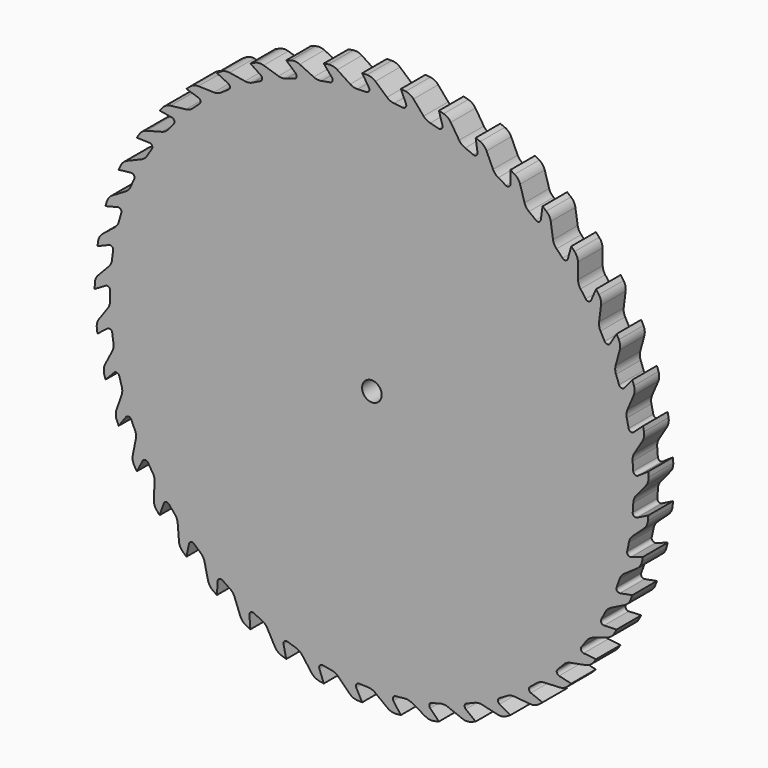
from build123d import *

# Parameters (mm, degrees)
F0_R            = 45
F1_DEPTH        = 5
F4_DEPTH        = 25
F4_COPIES_COUNT = 45
F5_R            = 2
F6_R            = 0.5
F7_R            = 1.5875
F8_DEPTH        = 25


# Not quite as in the source:
# - a pattern or mirror of a feature is missing from the dataset's text; its kind, count and spacing are read off the source's solid


with BuildPart() as f1:
    # F0 (on Front) → F1 (new body)
    with BuildSketch(Plane.XZ):
        Circle(F0_R)
    extrude(amount=F1_DEPTH)

    # F2 (on face) → F4 (cut)
    with BuildSketch(Plane.XZ.offset(5)):
        with BuildLine():
            Line((-6.2627895432, 44.5620630934), (-2.9646501341, 42.396472136))
            ThreePointArc((-2.9646501341, 42.396472136), (-1.4832286099, 42.4741101483), (0, 42.5))
            Line((0, 42.5), (-1.5704773516, 44.9725872159))
            ThreePointArc((-1.5704773516, 44.9725872159), (-3.9220084236, 44.8287614141), (-6.2627895432, 44.5620630934))
        make_face()
    f4 = extrude(amount=-F4_DEPTH, mode=Mode.SUBTRACT)

    # F4_copies: F4 ×45 about axis
    f4_copies_axis = Axis((0, 0, 0), (0, 1, 0))
    for i in range(1, F4_COPIES_COUNT):
        add(f4.rotate(f4_copies_axis, i * 360 / F4_COPIES_COUNT), mode=Mode.SUBTRACT)

    # F5
    f5_edges = [f1.edges().sort_by_distance(p)[0] for p in [
        (-6.26279, -2.5, 44.562063),
        (-2.96465, -2.5, 42.396472),
        (0, -2.5, 45),
        (2.96465, -2.5, 42.396472),
        (6.26279, -2.5, 44.562063),
        (8.836247, -2.5, 41.571273),
        (12.403681, -2.5, 43.256776),
        (14.535856, -2.5, 39.936936),
        (18.303149, -2.5, 41.109546),
        (19.952541, -2.5, 37.525273),
        (23.846367, -2.5, 38.162164),
        (24.980873, -2.5, 34.383222),
        (28.925442, -2.5, 34.472),
        (29.522981, -2.5, 30.571942),
        (33.441517, -2.5, 30.110877),
        (33.490457, -2.5, 26.165613),
        (37.306691, -2.5, 25.163681),
        (36.80608, -2.5, 21.25),
        (40.445732, -2.5, 19.726702),
        (39.405314, -2.5, 15.92078),
        (42.797543, -2.5, 13.905765),
        (41.237568, -2.5, 10.281681),
        (44.316349, -2.5, 7.814168),
        (42.267181, -2.5, 4.44246),
        (44.972587, -2.5, 1.570477),
        (42.47411, -2.5, -1.483229),
        (44.753485, -2.5, -4.703781),
        (41.85433, -2.5, -7.380048),
        (43.663308, -2.5, -10.886485),
        (40.419902, -2.5, -13.133222),
        (41.723273, -2.5, -16.857297),
        (38.198747, -2.5, -18.630774),
        (38.971143, -2.5, -22.5),
        (35.234097, -2.5, -23.765698),
        (35.460484, -2.5, -27.704766),
        (31.583655, -2.5, -28.438051),
        (31.259627, -2.5, -32.370291),
        (27.318473, -2.5, -32.556889),
        (26.450336, -2.5, -36.405765),
        (22.521569, -2.5, -36.042044),
        (21.12622, -2.5, -39.732642),
        (17.286307, -2.5, -38.825682),
        (15.390906, -2.5, -42.286168),
        (11.714588, -2.5, -40.853622),
        (9.356026, -2.5, -44.016642),
        (5.914857, -2.5, -42.086393),
        (3.139041, -2.5, -44.890382),
        (0, -2.5, -42.5),
        (-3.139041, -2.5, -44.890382),
        (-5.914857, -2.5, -42.086393),
        (-9.356026, -2.5, -44.016642),
        (-11.714588, -2.5, -40.853622),
        (-15.390906, -2.5, -42.286168),
        (-17.286307, -2.5, -38.825682),
        (-21.12622, -2.5, -39.732642),
        (-22.521569, -2.5, -36.042044),
        (-26.450336, -2.5, -36.405765),
        (-27.318473, -2.5, -32.556889),
        (-31.259627, -2.5, -32.370291),
        (-31.583655, -2.5, -28.438051),
        (-35.460484, -2.5, -27.704766),
        (-35.234097, -2.5, -23.765698),
        (-38.971143, -2.5, -22.5),
        (-38.198747, -2.5, -18.630774),
        (-41.723273, -2.5, -16.857297),
        (-40.419902, -2.5, -13.133222),
        (-43.663308, -2.5, -10.886485),
        (-41.85433, -2.5, -7.380048),
        (-44.753485, -2.5, -4.703781),
        (-42.47411, -2.5, -1.483229),
        (-44.972587, -2.5, 1.570477),
        (-42.267181, -2.5, 4.44246),
        (-44.316349, -2.5, 7.814168),
        (-41.237568, -2.5, 10.281681),
        (-42.797543, -2.5, 13.905765),
        (-39.405314, -2.5, 15.92078),
        (-40.445732, -2.5, 19.726702),
        (-36.80608, -2.5, 21.25),
        (-37.306691, -2.5, 25.163681),
        (-33.490457, -2.5, 26.165613),
        (-33.441517, -2.5, 30.110877),
        (-29.522981, -2.5, 30.571942),
        (-28.925442, -2.5, 34.472),
        (-24.980873, -2.5, 34.383222),
        (-23.846367, -2.5, 38.162164),
        (-19.952541, -2.5, 37.525273),
        (-18.303149, -2.5, 41.109546),
        (-14.535856, -2.5, 39.936936),
        (-12.403681, -2.5, 43.256776),
        (-8.836247, -2.5, 41.571273),
    ]]
    fillet(f5_edges, radius=F5_R)

    # F6
    f6_edges = [f1.edges().sort_by_distance(p)[0] for p in [
        (0, -2.5, 42.5),
        (-5.914857, -2.5, 42.086393),
        (5.914857, -2.5, 42.086393),
        (-11.714588, -2.5, 40.853622),
        (11.714588, -2.5, 40.853622),
        (-17.286307, -2.5, 38.825682),
        (17.286307, -2.5, 38.825682),
        (-22.521569, -2.5, 36.042044),
        (22.521569, -2.5, 36.042044),
        (-27.318473, -2.5, 32.556889),
        (27.318473, -2.5, 32.556889),
        (-31.583655, -2.5, 28.438051),
        (31.583655, -2.5, 28.438051),
        (-35.234097, -2.5, 23.765698),
        (35.234097, -2.5, 23.765698),
        (-38.198747, -2.5, 18.630774),
        (38.198747, -2.5, 18.630774),
        (-40.419902, -2.5, 13.133222),
        (40.419902, -2.5, 13.133222),
        (-41.85433, -2.5, 7.380048),
        (41.85433, -2.5, 7.380048),
        (-42.47411, -2.5, 1.483229),
        (42.47411, -2.5, 1.483229),
        (-42.267181, -2.5, -4.44246),
        (42.267181, -2.5, -4.44246),
        (-41.237568, -2.5, -10.281681),
        (41.237568, -2.5, -10.281681),
        (-39.405314, -2.5, -15.92078),
        (39.405314, -2.5, -15.92078),
        (-36.80608, -2.5, -21.25),
        (36.80608, -2.5, -21.25),
        (-33.490457, -2.5, -26.165613),
        (33.490457, -2.5, -26.165613),
        (-29.522981, -2.5, -30.571942),
        (29.522981, -2.5, -30.571942),
        (-24.980873, -2.5, -34.383222),
        (24.980873, -2.5, -34.383222),
        (-19.952541, -2.5, -37.525273),
        (19.952541, -2.5, -37.525273),
        (-14.535856, -2.5, -39.936936),
        (14.535856, -2.5, -39.936936),
        (-8.836247, -2.5, -41.571273),
        (8.836247, -2.5, -41.571273),
        (-2.96465, -2.5, -42.396472),
        (2.96465, -2.5, -42.396472),
    ]]
    fillet(f6_edges, radius=F6_R)

    # F7 (on face) → F8 (cut)
    with BuildSketch(Plane.XZ.offset(5)):
        Circle(F7_R)
    extrude(amount=-F8_DEPTH, mode=Mode.SUBTRACT)


solid = f1.part
